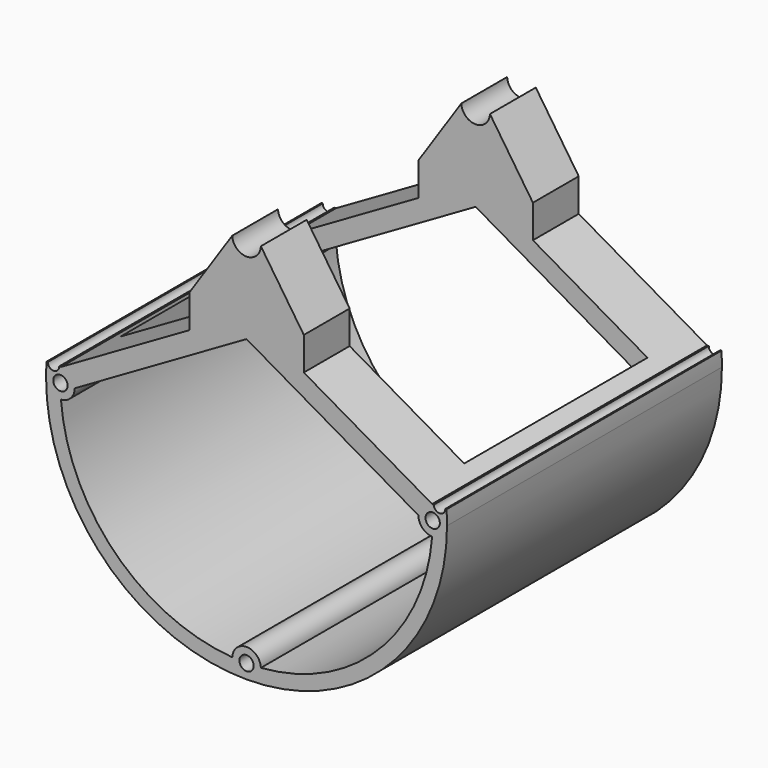
from build123d import *

# Parameters (mm, degrees)
F1_DEPTH  = 152.4
F2_R      = 3.175
F3_DEPTH  = 152.401
F5_DEPTH  = 152.401
F6_R      = 2.54
F7_DEPTH  = 152.401
F8_DEPTH  = 152.4
F9_W      = 152.4
F9_H      = 101.6
F10_DEPTH = 82.3067692308


# Not quite as in the source:
# - a feature names something its author has since deleted; it is built from what else it names


with BuildPart() as f1:
    # F0 (on Front) → F1 (new body)
    with BuildSketch(Plane.XZ):
        with BuildLine():
            ThreePointArc((-2.11e-07, -88.9), (62.8617927729, -62.8617929221), (88.9, 0))
            ThreePointArc((88.9, 0), (62.8617928475, 62.8617928475), (0, 88.9))
            ThreePointArc((0, 88.9), (-62.8617927742, 62.8617929208), (-88.9, 2.073e-07))
            ThreePointArc((-88.9, 2.073e-07), (-62.8617929954, -62.8617926996), (-2.11e-07, -88.9))
        make_face()
    extrude(amount=-F1_DEPTH)

    # F2 (on face) → F3 (cut, through all)
    with BuildSketch(Plane.XZ):
        with Locations((0, -82.55)):
            Circle(F2_R)
        with Locations((82.55, 0)):
            Circle(F2_R)
        with Locations((-82.55, 0)):
            Circle(F2_R)
    extrude(amount=-F3_DEPTH, mode=Mode.SUBTRACT)

    # F4 (on face) → F5 (cut, through all)
    with BuildSketch(Plane.XZ):
        Polygon((-94.202041626, 6.35), (0, 6.35), (132.5988769531, 6.35), (114.2803505063, 107.1024313569), (-94.202041626, 107.1024313569), align=None)
    extrude(amount=-F5_DEPTH, mode=Mode.SUBTRACT)

    # F6 (on face) + F2 (on face) → F7 (cut, through all)
    with BuildSketch(Plane.XZ):
        with Locations((-85.598, 6.35)):
            Circle(F6_R)
        with BuildLine():
            ThreePointArc((88.138, 6.35), (85.598, 8.89), (83.058, 6.35))
            ThreePointArc((83.058, 6.35), (85.598, 3.81), (88.138, 6.35))
        make_face()
    with BuildSketch(Plane.XZ):
        with BuildLine():
            Line((0, 43.9940905122), (-76.2, 0))
            ThreePointArc((-76.2, 0), (-77.974338005, -4.4029328075), (-82.3057692308, -6.3453015162))
            ThreePointArc((-82.3057692308, -6.3453015162), (-58.3716647869, -58.3716647869), (-6.3453015162, -82.3057692308))
            ThreePointArc((-6.3453015162, -82.3057692308), (0, -76.2), (6.3453015162, -82.3057692308))
            ThreePointArc((6.3453015162, -82.3057692308), (58.3716647869, -58.3716647869), (82.3057692308, -6.3453015162))
            ThreePointArc((82.3057692308, -6.3453015162), (77.974338005, -4.4029328075), (76.2, 0))
            Line((76.2, 0), (0, 43.9940905122))
        make_face()
    extrude(amount=-F7_DEPTH, mode=Mode.SUBTRACT)

    # F2 (on face) → F8 (join)
    with BuildSketch(Plane.XZ):
        with BuildLine():
            Line((0, 53.8645595374), (-25.4, 53.8645595374))
            Line((-25.4, 53.8645595374), (-25.4, 39.1998627))
            Line((-25.4, 39.1998627), (-82.3057692308, 6.3453015162))
            ThreePointArc((-82.3057692308, 6.3453015162), (-77.974338005, 4.4029328075), (-76.2, 0))
            Line((-76.2, 0), (0, 43.9940905122))
            Line((0, 43.9940905122), (76.2, 0))
            ThreePointArc((76.2, 0), (77.974338005, 4.4029328075), (82.3057692308, 6.3453015162))
            Line((82.3057692308, 6.3453015162), (25.4, 39.1998627))
            Line((25.4, 39.1998627), (25.4, 53.8645595374))
            Line((25.4, 53.8645595374), (0, 53.8645595374))
        make_face()
        with BuildLine():
            ThreePointArc((6.3453015162, 82.3057692308), (0, 76.2), (-6.3453015162, 82.3057692308))
            Line((-6.3453015162, 82.3057692308), (-25.4, 53.8645595374))
            Line((-25.4, 53.8645595374), (0, 53.8645595374))
            Line((0, 53.8645595374), (25.4, 53.8645595374))
            Line((25.4, 53.8645595374), (6.3453015162, 82.3057692308))
        make_face()
    extrude(amount=-F8_DEPTH)

    # F9 (on Top) → F10 (cut, through all)
    with BuildSketch(Plane.XY):
        with Locations((0, 76.2)):
            Rectangle(F9_W, F9_H)
    extrude(amount=F10_DEPTH, mode=Mode.SUBTRACT)


solid = f1.part
